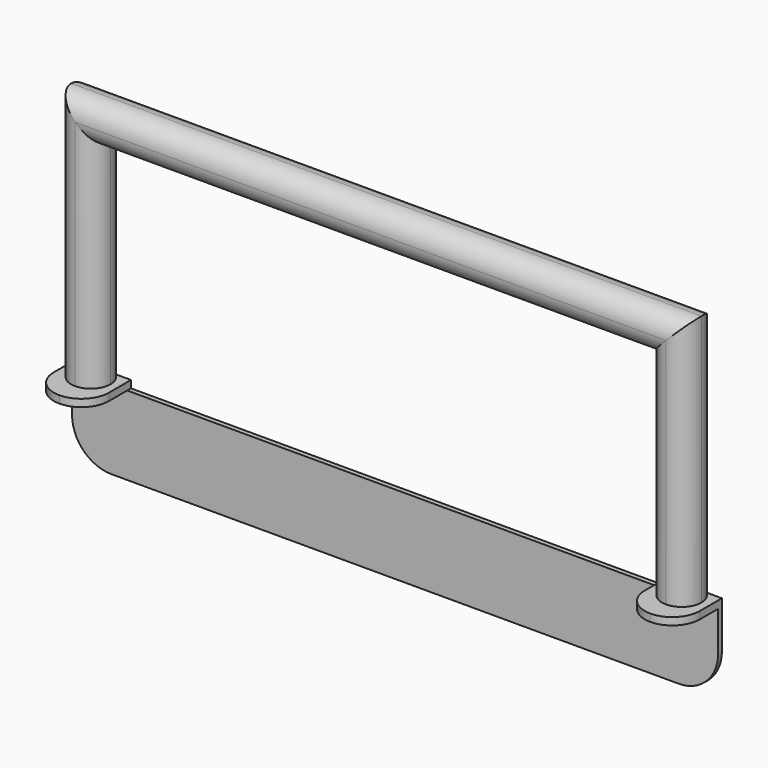
from build123d import *

# Parameters (mm, degrees)
F2_DEPTH = 5
F3_R     = 2.49999
F4_W     = 80
F4_H     = 32
F5_DEPTH = 0.5
F7_DEPTH = 7
F8_DEPTH = 0.6
F9_R     = 3.49999
F10_R    = 5


# Not quite as in the source:
# - a fillet or chamfer is up to 0.001 mm smaller than in the source, because OpenCascade refuses the exact size


with BuildPart() as f2:
    # F1 (on Front) → F2 (new body)
    with BuildSketch(Plane.XZ):
        Polygon((-40, 32), (-40, 0), (-35, 0), (-35, 27), (35, 27), (35, 0), (40, 0), (40, 32), align=None)
    extrude(amount=F2_DEPTH)

    # F3 (radius 2.5 in the source; OpenCascade refuses exactly that, so slightly less here)
    f3_edges = [f2.edges().sort_by_distance(p)[0] for p in [
        (-35, -5, 13.5),
        (-35, 0, 13.5),
        (40, -5, 16),
        (40, 0, 16),
        (35, -5, 13.5),
        (35, 0, 13.5),
        (0, 0, 27),
        (0, 0, 32),
        (-40, 0, 16),
        (0, -5, 32),
        (-40, -5, 16),
        (0, -5, 27),
    ]]
    fillet(f3_edges, radius=F3_R)

    # F4 (on Front) → F5 (cut)
    with BuildSketch(Plane.XZ):
        with Locations((0, 16)):
            Rectangle(F4_W, F4_H)
    extrude(amount=F5_DEPTH, mode=Mode.SUBTRACT)

    # F6 (on face) → F7 (join)
    with BuildSketch(Plane(origin=(0, -0.5, 0), x_dir=(-1, 0, 0), z_dir=(0, 1, 0))):
        Polygon((-35.9999933333, 0), (-37.5, 0), (-39.0000066667, 0), (-41, 0), (-41, -0.936), (-34, -0.936), (-34, 0), align=None)
        Polygon((41, 0), (39.0000066667, 0), (37.5, 0), (35.9999933333, 0), (34, 0), (34, -0.936), (41, -0.936), align=None)
    extrude(amount=-F7_DEPTH)

    # F6 (on face) → F8 (join)
    with BuildSketch(Plane(origin=(0, -0.5, 0), x_dir=(-1, 0, 0), z_dir=(0, 1, 0))):
        Polygon((-34, -0.936), (-41, -0.936), (-41, -10.936), (0, -10.936), (41, -10.936), (41, -0.936), (34, -0.936), (0, -0.936), align=None)
    extrude(amount=-F8_DEPTH)

    # F9 (radius 3.5 in the source; OpenCascade refuses exactly that, so slightly less here)
    f9_edges = [f2.edges().sort_by_distance(p)[0] for p in [
        (41, -7.5, -0.468),
        (34, -7.5, -0.468),
        (-34, -7.5, -0.468),
        (-41, -7.5, -0.468),
    ]]
    fillet(f9_edges, radius=F9_R)

    # F10
    f10_edges = [f2.edges().sort_by_distance(p)[0] for p in [
        (41, -0.8, -10.936),
        (-41, -0.8, -10.936),
    ]]
    fillet(f10_edges, radius=F10_R)


solid = f2.part
